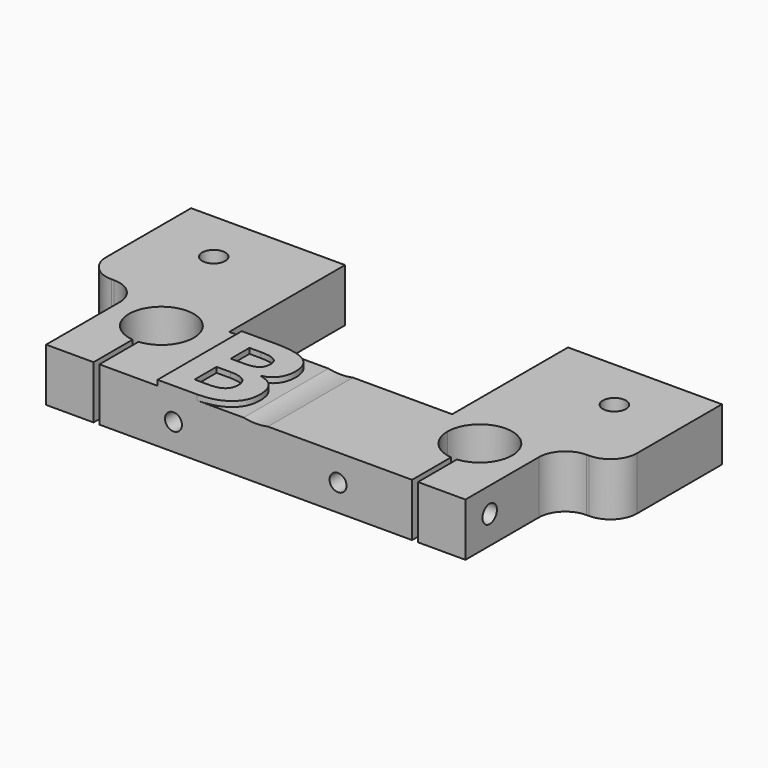
from build123d import *

# Parameters (mm, degrees)
F1_DEPTH      = 10
F2_R          = 1.6
F2_R_2        = 10.75
F3_DEPTH      = 47.2759499461
F4_R          = 2.175
F5_DEPTH      = 10.001
F6_R          = 5
F7_R          = 5
F8_R          = 1.4
F9_DEPTH      = 18
F8_R_2        = 1.7
F10_DEPTH     = 8.947754083
F12_TEXT_SIZE = 27.7777777778
F13_DEPTH     = 1


# Not quite as in the source:
# - Text() gives the source's letters only with a copy of the font that has no kerning and outlines rounded to 1/6400 em; it was checked with that copy


with BuildPart() as f1:
    # F0 (on Top) → F1 (new body)
    with BuildSketch(Plane.XY):
        Polygon((-39.5, -13.8158900663), (0, -13.8158900663), (0, 6.1841099337), (-21, 6.1841099337), (-21, 33.4590598798), (-50, 33.4590598798), (-50, 8.4590598798), (-39.5, 8.4590598798), align=None)
    extrude(amount=F1_DEPTH)

    # F2 (on face) → F3 (cut, through all)
    with BuildSketch(Plane.XZ.offset(13.8158900663)):
        with Locations((-15.5, 5)):
            Circle(F2_R)
        with Locations((0, 20.5)):
            Circle(F2_R_2)
    extrude(amount=-F3_DEPTH, mode=Mode.SUBTRACT)

    # F4 (on face) → F5 (cut, through all)
    with BuildSketch(Plane.XY.offset(10)):
        with BuildLine():
            ThreePointArc((-29.446754083, -4.6157997034), (-25.4952913472, -2.6540411344), (-23.9, 1.4590598798))
            ThreePointArc((-23.9, 1.4590598798), (-34.1131010142, 5.9637685326), (-30.553245917, -4.6157997034))
            Line((-30.553245917, -4.6157997034), (-30.553245917, -1.6342723975))
            Line((-30.553245917, -1.6342723975), (-29.446754083, -1.6342723975))
            Line((-29.446754083, -1.6342723975), (-29.446754083, -4.6157997034))
        make_face()
        with BuildLine():
            Line((-30.553245917, -1.6342723975), (-30.553245917, -4.6157997034))
            ThreePointArc((-30.553245917, -4.6157997034), (-30, -4.6409401202), (-29.446754083, -4.6157997034))
            Line((-29.446754083, -4.6157997034), (-29.446754083, -1.6342723975))
            Line((-29.446754083, -1.6342723975), (-30.553245917, -1.6342723975))
        make_face()
        with BuildLine():
            ThreePointArc((-29.446754083, -4.6157997034), (-30, -4.6409401202), (-30.553245917, -4.6157997034))
            Line((-30.553245917, -4.6157997034), (-30.553245917, -14.7385904565))
            Line((-30.553245917, -14.7385904565), (-29.446754083, -14.7385904565))
            Line((-29.446754083, -14.7385904565), (-29.446754083, -4.6157997034))
        make_face()
        with Locations((-37.7414673567, 23.4590598798)):
            Circle(F4_R)
    extrude(amount=-F5_DEPTH, mode=Mode.SUBTRACT)

    # F6
    f6_edges = [f1.edges().sort_by_distance(p)[0] for p in [
        (-50, 8.45906, 5),
    ]]
    fillet(f6_edges, radius=F6_R)

    # F7
    f7_edges = [f1.edges().sort_by_distance(p)[0] for p in [
        (-39.5, 8.45906, 5),
    ]]
    fillet(f7_edges, radius=F7_R)

    # F8 (on face) → F9 (cut)
    with BuildSketch(Plane(origin=(-39.5, 0, 0), x_dir=(0, -1, 0), z_dir=(-1, 0, 0))):
        with Locations((8.1005264074, 5.3087547421)):
            Circle(F8_R)
    extrude(amount=-F9_DEPTH, mode=Mode.SUBTRACT)

    # F8 (on face) → F10 (cut, through all)
    with BuildSketch(Plane(origin=(-39.5, 0, 0), x_dir=(0, -1, 0), z_dir=(-1, 0, 0))):
        with Locations((8.1005264074, 5.3087547421)):
            Circle(F8_R_2)
        with Locations((8.1005264074, 5.3087547421)):
            Circle(F8_R, mode=Mode.SUBTRACT)
        with Locations((8.1005264074, 5.3087547421)):
            Circle(F8_R)
    extrude(amount=-F10_DEPTH, mode=Mode.SUBTRACT)

    # F11: F1 across plane


with BuildPart() as f1_1:
    add(f1.part)
    add(f1.part.mirror(Plane.YZ))

    # F12 (on face) → F13 (join)
    with BuildSketch(Plane.XY.offset(10)):
        with Locations((-21, -13.8158900663)):
            Text('B', F12_TEXT_SIZE, font='Open Sans', font_style=FontStyle.BOLD, text_align=(TextAlign.LEFT, TextAlign.BOTTOM))
    extrude(amount=F13_DEPTH)


solid = f1_1.part
